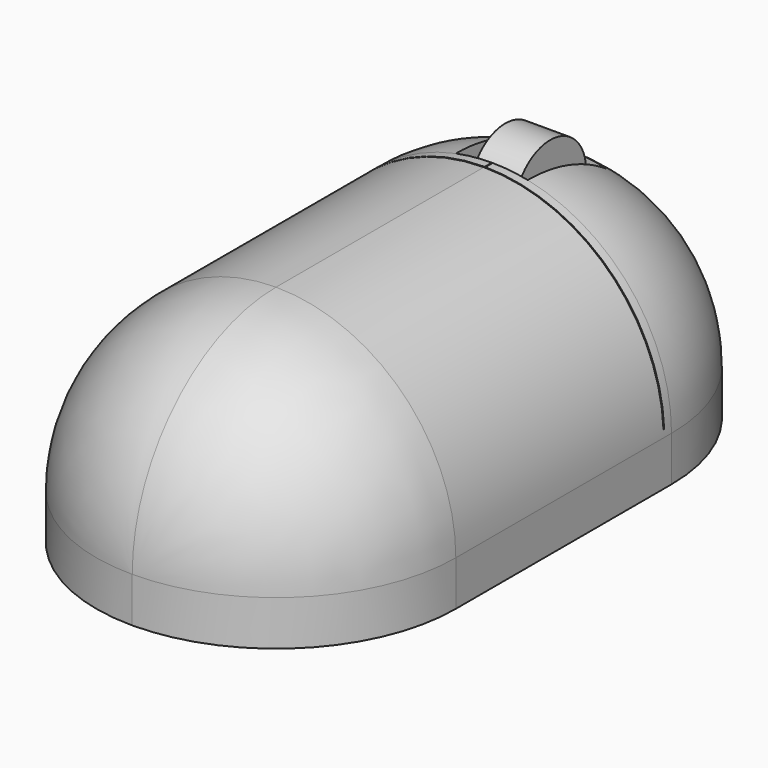
from build123d import *

# Parameters (mm, degrees)
F2_DEPTH    = 31.75
F3_DEPTH    = 7.62
F4_R        = 6.35
F5_DEPTH    = 3.175
F6_DEPTH    = 3.175
F7_T1_DEPTH = 127
F7_T4_ANGLE = 180
F12_W       = 50.8
F12_H       = 24.638
F13_DEPTH   = 0.127
F16_W       = 29.0950196795
F16_H       = 29.9766859971
F17_DEPTH   = 0.127
F19_R       = 25.39999


# Not quite as in the source:
# - a fillet or chamfer that OpenCascade refuses, or shapes differently, is made with other operations: its cross-section is extruded or revolved along the edge and cut away or added
# - a fillet or chamfer is up to 0.001 mm smaller than in the source, because OpenCascade refuses the exact size


with BuildPart() as f2:
    # F1 (on Top) → F2 (new body)
    with BuildSketch(Plane.XY):
        with BuildLine():
            ThreePointArc((25.4, 0), (0, 25.4), (-25.4, 0))
            Line((-25.4, 0), (0, 0))
            Line((0, 0), (25.4, 0))
        make_face()
        with BuildLine():
            ThreePointArc((25.4, 0), (0, -25.4), (-25.4, 0))
            Line((-25.4, 0), (-25.4, -63.5))
            Line((-25.4, -63.5), (25.4, -63.5))
            Line((25.4, -63.5), (25.4, 0))
        make_face()
        with BuildLine():
            Line((0, 0), (-25.4, 0))
            ThreePointArc((-25.4, 0), (0, -25.4), (25.4, 0))
            Line((25.4, 0), (0, 0))
        make_face()
    extrude(amount=-F2_DEPTH)

    # F0 (on Top) → F3 (cut)
    with BuildSketch(Plane.XY):
        Polygon((5.08, 13.97), (-5.08, 13.97), (-5.08, 0), (0, 0), (5.08, 0), align=None)
    extrude(amount=-F3_DEPTH, mode=Mode.SUBTRACT)

    # F7: fillet of radius 25.4 on 3 edges, made by hand

    # F7_s2 → F7_t1 (cut)
    with BuildSketch(Plane.XZ):
        with BuildLine():
            ThreePointArc((25.4, -25.4), (17.9605122421, -7.4394877579), (0, 0))
            Line((0, 0), (25.4, 0))
            Line((25.4, 0), (25.4, -25.4))
        make_face()
        with BuildLine():
            ThreePointArc((-25.4, -25.4), (-17.9605122421, -7.4394877579), (0, 0))
            Line((0, 0), (-25.4, 0))
            Line((-25.4, 0), (-25.4, -25.4))
        make_face()
    extrude(amount=F7_T1_DEPTH, mode=Mode.SUBTRACT)

    # F7_s3 → F7_t4 (revolve, cut)
    with BuildSketch(Plane.XZ):
        with BuildLine():
            ThreePointArc((25.4, -25.4), (17.9605122421, -7.4394877579), (0, 0))
            Line((0, 0), (25.4, 0))
            Line((25.4, 0), (25.4, -25.4))
        make_face()
    revolve(axis=Axis((0, 0, 0), (0, 0, 1)), revolution_arc=F7_T4_ANGLE, mode=Mode.SUBTRACT)


with BuildPart() as f5:
    # F4 (on Right) → F5 (new body)
    with BuildSketch(Plane.YZ):
        Circle(F4_R)
    extrude(amount=F5_DEPTH)

    # F4 (on Right) → F6 (join)
    with BuildSketch(Plane.YZ):
        Circle(F4_R)
    extrude(amount=-F6_DEPTH)


with BuildPart() as f2_1:
    # F8: moved
    add(f2.part.moved(Location((0, -6.35, 0))))


with BuildPart() as f5_1:
    # F10: moved
    add(f5.part.moved(Location((0, 0, -5.08))))


with BuildPart() as f13:
    # F12 (on offset) → F13 (new body)
    with BuildSketch(Plane.XZ.offset(6.35)):
        with Locations((0.0398121774, -12.0800452944)):
            Rectangle(F12_W, F12_H)
    extrude(amount=F13_DEPTH)


with BuildPart() as f13_1:
    # F14: moved
    add(f13.part.moved(Location((0, -1.27, 0))))


with BuildPart() as f2_2:
    add(f2_1.part)

    # F15: cut F13
    add(f13_1.part, mode=Mode.SUBTRACT)


with BuildPart() as f17:
    # F16 (on Right) → F17 (new body)
    with BuildSketch(Plane.YZ):
        with Locations((7.0028568152, -9.0095989872)):
            Rectangle(F16_W, F16_H)
    extrude(amount=F17_DEPTH)


with BuildPart() as f2_3:
    add(f2_2.part)

    # F18: cut F17
    add(f17.part, mode=Mode.SUBTRACT)

    # F19 (radius 25.4 in the source; OpenCascade refuses exactly that, so slightly less here)
    f19_edges = [f2_3.edges().sort_by_distance(p)[0] for p in [
        (-17.960512, -69.85, -7.439488),
        (-25.4, -69.85, -28.575),
        (25.4, -69.85, -28.575),
        (17.960512, -69.85, -7.439488),
    ]]
    fillet(f19_edges, radius=F19_R)


solid = Compound([f5_1.part, f2_3.part])
